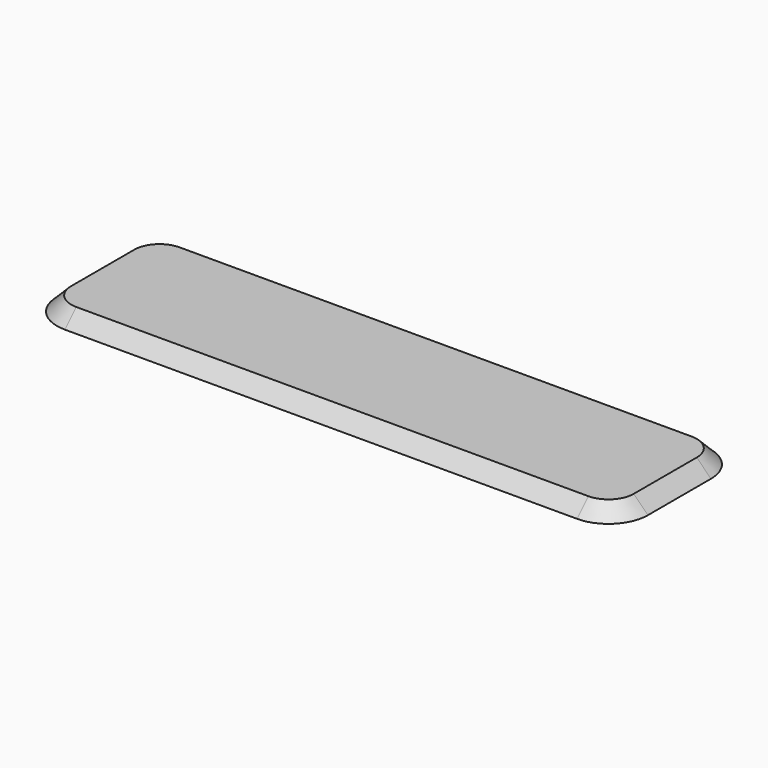
from build123d import *

# Parameters (mm, degrees)
F0_W     = 75
F0_H     = 20
F1_DEPTH = 1.8
F2_R     = 5
F3_SIZE  = 1.79999


# Not quite as in the source:
# - a fillet or chamfer is up to 0.001 mm smaller than in the source, because OpenCascade refuses the exact size


with BuildPart() as f1:
    # F0 (on Top) → F1 (new body)
    with BuildSketch(Plane.XY):
        Rectangle(F0_W, F0_H)
    extrude(amount=F1_DEPTH)

    # F2
    f2_edges = [f1.edges().sort_by_distance(p)[0] for p in [
        (-37.5, -10, 0.9),
        (-37.5, 10, 0.9),
        (37.5, -10, 0.9),
        (37.5, 10, 0.9),
    ]]
    fillet(f2_edges, radius=F2_R)

    # F3 (size 1.8 in the source; OpenCascade refuses exactly that, so slightly less here)
    f3_edges = [f1.edges().sort_by_distance(p)[0] for p in [
        (0, -10, 1.8),
        (-36.035534, -8.535534, 1.8),
        (36.035534, -8.535534, 1.8),
        (-37.5, 0, 1.8),
        (37.5, 0, 1.8),
        (-36.035534, 8.535534, 1.8),
        (36.035534, 8.535534, 1.8),
        (0, 10, 1.8),
    ]]
    chamfer(f3_edges, length=F3_SIZE)


solid = f1.part
